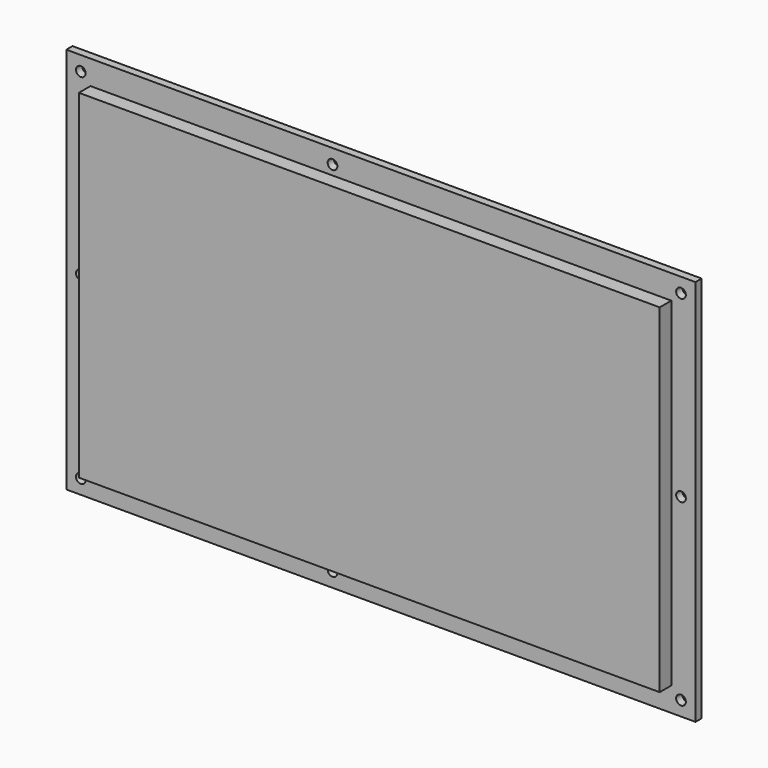
from build123d import *

# Parameters (mm, degrees)
F0_W     = 120
F0_H     = 70
F2_DEPTH = 3
F1_W     = 130
F1_H     = 80
F3_DEPTH = 1.6
F4_D     = 2


# Not quite as in the source:
# - a feature names something its author has since deleted; it is built from what else it names


with BuildPart() as f2:
    # F0 (on Front) → F2 (new body)
    with BuildSketch(Plane.XZ):
        Rectangle(F0_W, F0_H)
    extrude(amount=F2_DEPTH)

    # F1 (on Front) → F3 (join)
    with BuildSketch(Plane.XZ):
        Rectangle(F1_W, F1_H)
    extrude(amount=-F3_DEPTH)

    # F4 (through all)
    with Locations(Plane.XZ):
        with Locations((62, 37), (62, 0), (62, -37), (-62, 37), (-62, 0), (-62, -37), (-10, 37), (-10, -37)):
            Hole(F4_D / 2)


solid = f2.part
